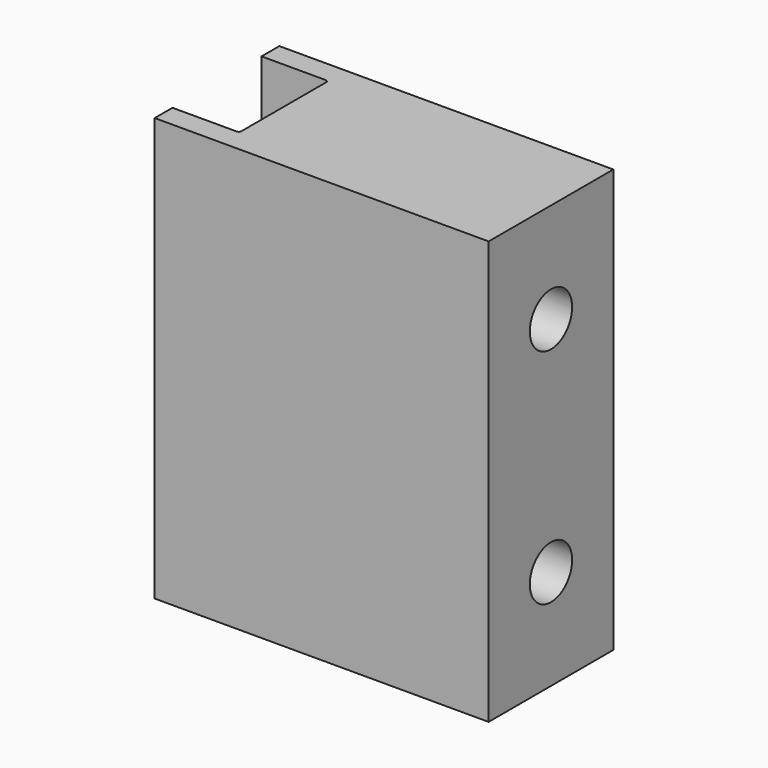
from build123d import *

# Parameters (mm, degrees)
F1_DEPTH       = 120.65
F3_D           = 20.6375
F3_CBORE_D     = 30.1752
F3_CBORE_DEPTH = 28.448
F4_R           = 1.524


# Not quite as in the source:
# - a length typed as a fraction of an inch, garbled in the dataset ("3 / 203.2 mm" for 3/8 in), is restored


with BuildPart() as f1:
    # F0 (on Top) → F1 (new body, symmetric)
    with BuildSketch(Plane.XY):
        Polygon((95.25, 44.45), (-95.25, 44.45), (-95.25, 31.75), (-57.15, 31.75), (-57.15, -31.75), (-95.25, -31.75), (-95.25, -44.45), (95.25, -44.45), align=None)
    extrude(amount=F1_DEPTH, both=True)

    # F3 (through all)
    with Locations(Plane.YZ.offset(95.25)):
        with Locations((0, 63.5), (0, -63.5)):
            CounterBoreHole(F3_D / 2, F3_CBORE_D / 2, F3_CBORE_DEPTH)

    # F4
    f4_edges = [f1.edges().sort_by_distance(p)[0] for p in [
        (-57.15, -31.75, 0),
        (-57.15, 31.75, 0),
    ]]
    fillet(f4_edges, radius=F4_R)


solid = f1.part
